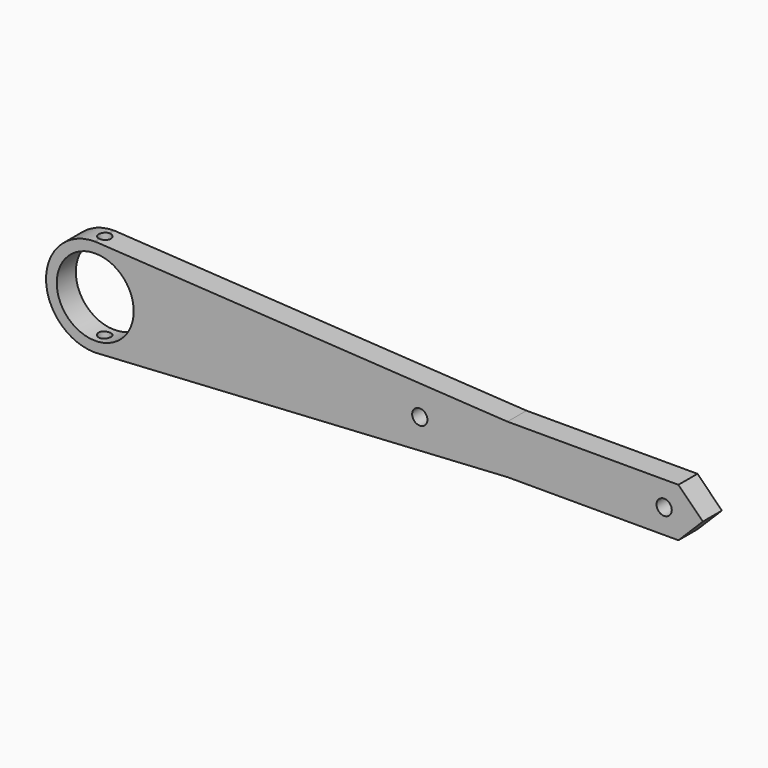
from build123d import *

# Parameters (mm, degrees)
F0_R     = 16.002
F0_R_2   = 3.175
F1_DEPTH = 9.906
F3_R     = 16.002
F3_R_2   = 3.175
F4_DEPTH = 9.906
F6_SIZE  = 10.15999
F7_R     = 2.54
F8_DEPTH = 63.5


# Not quite as in the source:
# - a fillet or chamfer is up to 0.001 mm smaller than in the source, because OpenCascade refuses the exact size


with BuildPart() as f1:
    # F0 (on Front) → F1 (new body)
    with BuildSketch(Plane.XZ):
        with BuildLine():
            Line((-40.64, -10.16), (40.64, -10.16))
            Line((40.64, -10.16), (40.64, 10.16))
            Line((40.64, 10.16), (-40.64, 10.16))
            Line((-40.64, 10.16), (-212.09, 20.32))
            Line((-212.09, 20.32), (-212.3586240849, 20.32))
            ThreePointArc((-212.3586240849, 20.32), (-225.7918722454, 15.1275163151), (-232.41, 2.3363307568))
            Line((-232.41, 2.3363307568), (-232.41, -2.3363307568))
            ThreePointArc((-232.41, -2.3363307568), (-225.7918722455, -15.1275163151), (-212.3586240849, -20.32))
            Line((-212.3586240849, -20.32), (-212.09, -20.32))
            Line((-212.09, -20.32), (-40.64, -10.16))
        make_face()
        with Locations((-212.09, 0)):
            Circle(F0_R, mode=Mode.SUBTRACT)
        with Locations((-77.089, 0)):
            Circle(F0_R_2, mode=Mode.SUBTRACT)
        with Locations((24.5364, 0)):
            Circle(F0_R_2, mode=Mode.SUBTRACT)
        with BuildLine():
            ThreePointArc((-212.3586240849, -20.32), (-212.2243120425, -20.320443886), (-212.09, -20.32))
            Line((-212.09, -20.32), (-212.3586240849, -20.32))
        make_face()
        with BuildLine():
            Line((-212.3586240849, 20.32), (-212.09, 20.32))
            ThreePointArc((-212.09, 20.32), (-212.2243120425, 20.320443886), (-212.3586240849, 20.32))
        make_face()
        with BuildLine():
            ThreePointArc((-232.41, 2.3363307568), (-232.5447559285, 0), (-232.41, -2.3363307568))
            Line((-232.41, -2.3363307568), (-232.41, 2.3363307568))
        make_face()
    extrude(amount=F1_DEPTH)

    # F3 (on face) → F4 (join)
    with BuildSketch(Plane.XZ.offset(9.906)):
        with BuildLine():
            ThreePointArc((-212.09, 20.32), (-232.5447559285, 0), (-212.09, -20.32))
            Line((-212.09, -20.32), (-40.64, -10.16))
            Line((-40.64, -10.16), (40.64, -10.16))
            Line((40.64, -10.16), (40.64, 10.16))
            Line((40.64, 10.16), (-40.64, 10.16))
            Line((-40.64, 10.16), (-212.09, 20.32))
        make_face()
        with Locations((-212.09, 0)):
            Circle(F3_R, mode=Mode.SUBTRACT)
        with Locations((-77.089, 0)):
            Circle(F3_R_2, mode=Mode.SUBTRACT)
        with Locations((24.5364, 0)):
            Circle(F3_R_2, mode=Mode.SUBTRACT)
        Polygon((-192.0276897852, 9.9897326363), (-191.4355526853, 11.4626650533), (-190.8434155854, 12.9355974702), (-161.479297027, 1.1308576164), (-159.3415343892, 0.2714505221), (-138.9796634154, 8.3541679114), (-109.9172381334, 0.2630833417), (-106.984711484, 1.0945316722), (-104.048270324, 0.2770158067), (-101.1118291641, -0.5405000589), (-104.0443558136, -1.3719483894), (-106.976882463, -2.2033967199), (-109.913323623, -1.3858808543), (-138.9771856379, -9.6262491233), (-159.3452632945, -1.4380292869), (-161.4867548376, -2.2881020016), (-163.6245174754, -1.4286949073), (-165.7622801132, -0.5692878129), align=None, mode=Mode.SUBTRACT)
        Polygon((-157.2037717514, -0.5879565723), (-159.3452632945, -1.4380292869), (-138.9771856379, -9.6262491233), (-109.913323623, -1.3858808543), (-112.8497647829, -0.5683649888), (-138.8883433663, -7.9509859432), align=None)
        Polygon((-138.9796634154, 8.3541679114), (-159.3415343892, 0.2714505221), (-157.2037717514, -0.5879565723), (-138.8906361201, 6.6815080074), (-112.8497647829, -0.5683649888), (-109.9172381334, 0.2630833417), align=None)
        Polygon((-190.8434155854, 12.9355974702), (-191.4355526853, 11.4626650533), (-163.6207885701, 0.2807849018), (-161.479297027, 1.1308576164), align=None)
        Polygon((-163.6207885701, 0.2807849018), (-191.4355526853, 11.4626650533), (-192.0276897852, 9.9897326363), (-165.7622801132, -0.5692878129), align=None)
        Polygon((-106.9807969735, -0.5544325238), (-109.913323623, -1.3858808543), (-106.976882463, -2.2033967199), (-104.0443558136, -1.3719483894), align=None)
        Polygon((-112.8497647829, -0.5683649888), (-109.913323623, -1.3858808543), (-106.9807969735, -0.5544325238), (-109.9172381334, 0.2630833417), align=None)
        Polygon((-104.048270324, 0.2770158067), (-106.9807969735, -0.5544325238), (-104.0443558136, -1.3719483894), (-101.1118291641, -0.5405000589), align=None)
        Polygon((-106.984711484, 1.0945316722), (-109.9172381334, 0.2630833417), (-106.9807969735, -0.5544325238), (-104.048270324, 0.2770158067), align=None)
        Polygon((-161.479297027, 1.1308576164), (-163.6207885701, 0.2807849018), (-161.4830259323, -0.5786221926), (-159.3415343892, 0.2714505221), align=None)
        Polygon((-161.4830259323, -0.5786221926), (-163.6207885701, 0.2807849018), (-165.7622801132, -0.5692878129), (-163.6245174754, -1.4286949073), align=None)
        Polygon((-159.3415343892, 0.2714505221), (-161.4830259323, -0.5786221926), (-159.3452632945, -1.4380292869), (-157.2037717514, -0.5879565723), align=None)
        Polygon((-159.3452632945, -1.4380292869), (-161.4830259323, -0.5786221926), (-163.6245174754, -1.4286949073), (-161.4867548376, -2.2881020016), align=None)
    extrude(amount=-F4_DEPTH)

    # F6 (size 10.16 in the source; OpenCascade refuses exactly that, so slightly less here)
    f6_edges = [f1.edges().sort_by_distance(p)[0] for p in [
        (40.64, -4.953, -10.16),
        (40.64, -4.953, 10.16),
    ]]
    chamfer(f6_edges, length=F6_SIZE)

    # F7 (on Top) → F8 (cut, symmetric)
    with BuildSketch(Plane.XY):
        with Locations((-212.09, -4.953)):
            Circle(F7_R)
    extrude(amount=F8_DEPTH, both=True, mode=Mode.SUBTRACT)


solid = f1.part
